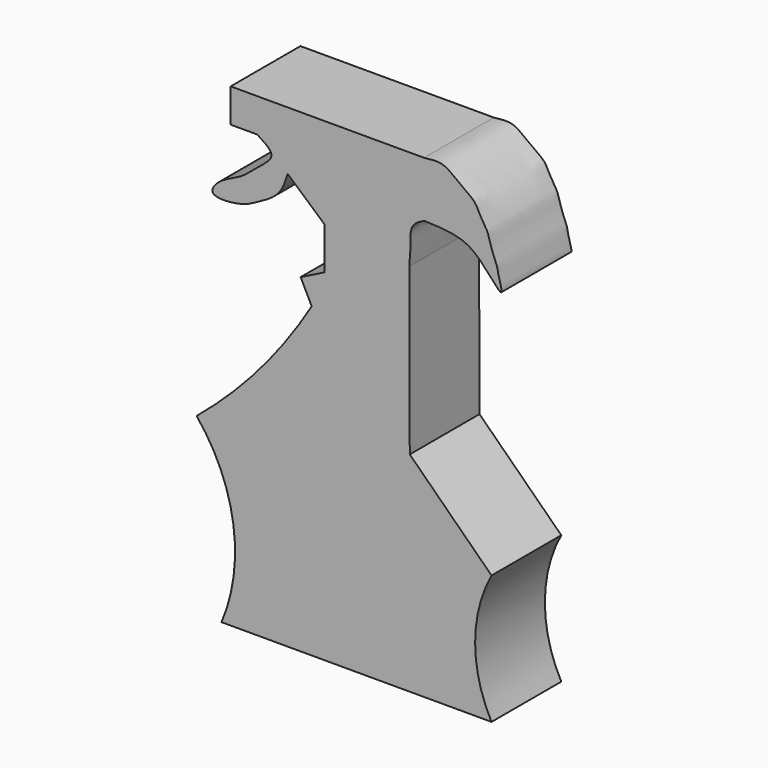
from build123d import *

# Parameters (mm, degrees)
F1_DEPTH = 25.4


with BuildPart() as f1:
    # F0 (on Front) → F1 (new body)
    with BuildSketch(Plane.XZ):
        with BuildLine():
            Line((22.6471498609, 56.1708956957), (-33.6727388203, 56.1708956957))
            Line((-33.6727388203, 56.1708956957), (-33.6727388203, 46.3372655213))
            Line((-33.6727388203, 46.3372655213), (-25.9174183011, 46.3372655213))
            add(Edge.make_bspline(
                [(-25.9174183011, 46.3372655213), (-23.8384248423, 45.0250805606), (-19.6311358124, 42.3695929412), (-26.4548745148, 37.7604244944), (-30.251269397, 33.7022554926), (-36.9185112274, 31.5489744559), (-40.9623640059, 25.8500064631), (-30.4127234084, 26.4631393418), (-26.2043699608, 28.9562646016), (-19.1149018323, 32.5915279181), (-17.7463418011, 36.9940384372), (-17.0775894076, 39.1453430057)],
                knots=[0, 0, 0, 0, 0.1069746269, 0.2164860944, 0.326296391, 0.4459968404, 0.5346841258, 0.6574790218, 0.7649065343, 0.8851206273, 1, 1, 1, 1], degree=3))
            Line((-17.0775894076, 39.1453430057), (-6.3435137272, 29.674096033))
            Line((-6.3435137272, 29.674096033), (-6.3435137272, 17.36147888))
            Line((-6.3435137272, 17.36147888), (-13.2890921086, 13.8886868954))
            Line((-13.2890921086, 13.8886868954), (-10.0688668171, 7.4482414939))
            ThreePointArc((-10.0688668171, 7.4482414939), (-25.1639599361, -13.4965769846), (-43.5970760882, -31.5732881427))
            ThreePointArc((-43.5970760882, -31.5732881427), (-32.8946720473, -55.8225948104), (-36.3357998431, -82.1043178439))
            Line((-36.3357998431, -82.1043178439), (42.3144139349, -82.1043178439))
            ThreePointArc((42.3144139349, -82.1043178439), (37.5371457467, -63.3268244565), (42.3144139349, -44.549331069))
            Line((42.3144139349, -44.549331069), (18.5016249106, -21.2456751615))
            Line((18.5016249106, -21.2456751615), (18.3543357998, 26.9130244851))
            add(Edge.make_bspline(
                [(22.6471498609, 40.027089417), (21.2792029286, 39.3295081026), (18.3426400433, 37.8320147795), (18.8097058732, 31.5486892751), (18.5016249106, 28.412426806), (18.3543357998, 26.9130244851)],
                knots=[0, 0, 0, 0, 0.3127842622, 0.6714519647, 1, 1, 1, 1], degree=3))
            add(Edge.make_bspline(
                [(22.6471498609, 56.1708956957), (24.6242757207, 56.4167795131), (28.4765464917, 56.8958643616), (32.1259487873, 53.3392921925), (37.4867669651, 50.1030116949), (38.4358992651, 47.6178089471), (40.751216997, 43.8553132507), (41.3864216625, 42.7681305631), (42.337306284, 38.8063167025), (44.181487922, 34.8741808016), (44.0560653004, 33.8002724839), (46.8419924844, 25.5814490103), (38.8226009812, 36.3773031204), (32.4243539132, 39.6728607383), (25.9777945234, 39.9064199647), (22.6471498609, 40.027089417)],
                knots=[0, 0, 0, 0, 0.0835853039, 0.1628592441, 0.2495253229, 0.3090454849, 0.3812735114, 0.4222536655, 0.4937216176, 0.5660430876, 0.6098018867, 0.6855943774, 0.7886561121, 0.8908082049, 1, 1, 1, 1], degree=3))
        make_face()
    extrude(amount=F1_DEPTH)


solid = f1.part
